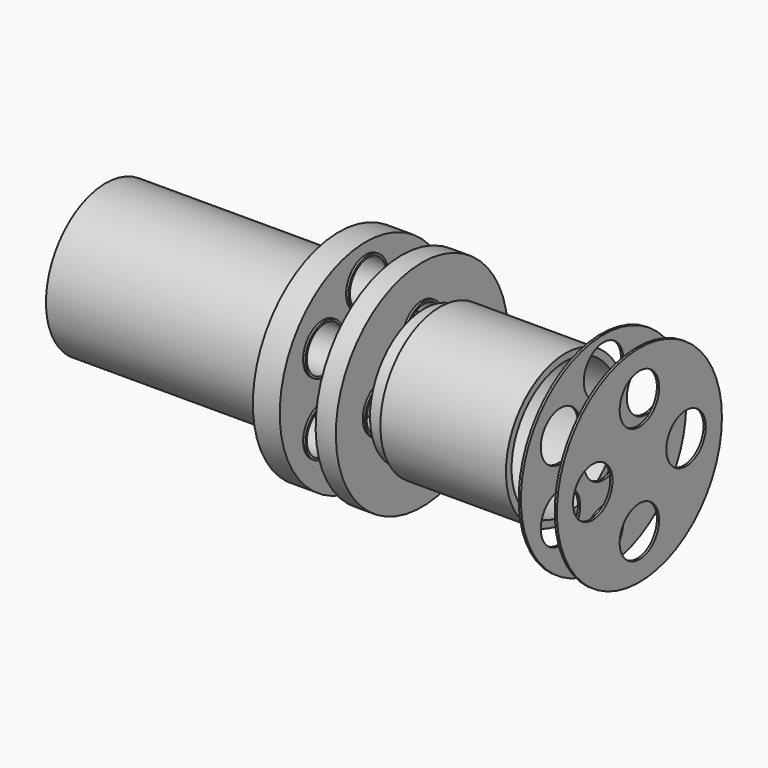
from build123d import *

# Parameters (mm, degrees)
F0_W            = 25.4
F0_H            = 47.9171
F2_R            = 52.9171
F2_R_2          = 47.9171
F3_DEPTH        = 152.4
F5_R            = 76.2
F5_R_2          = 17.4625
F7_DEPTH        = 1.5875
F8_R            = 76.2
F8_R_2          = 73.152
F9_DEPTH        = 17.4625
F10_R           = 73.152
F10_R_2         = 17.4625
F11_DEPTH       = 1.5875
F12_R           = 17.4625
F12_R_2         = 16.0655
F13_DEPTH       = 1.5875
F13_DEPTH_BACK  = 20.6375
F15_D           = 10.16
F15_CBORE_D     = 19.05
F15_CBORE_DEPTH = 12.7
F20_R           = 16.0655
F21_DEPTH       = 14.2875
F20_R_2         = 17.4625
F22_DEPTH       = 1.5875
F22_DEPTH_BACK  = 15.875
F23_W           = 88.9
F23_H           = 4.9784
F26_R           = 73.152
F26_R_2         = 17.4625
F27_DEPTH       = 1.5875
F29_R           = 73.025
F29_R_2         = 17.4625
F30_DEPTH       = 1.5875


# Not quite as in the source:
# - a length typed as a fraction of an inch, garbled in the dataset ("3 / 203.2 mm" for 3/8 in), is restored
# - a feature names something its author has since deleted; it is built from what else it names
# - the program builds the solid bodies; features that only make, move or delete a surface that nothing else refers to are left out


with BuildPart() as f1:
    # F0 (on Front) → F1 (revolve)
    with BuildSketch(Plane.XZ):
        with Locations((38.1, 23.95855)):
            Rectangle(F0_W, F0_H)
    revolve(axis=Axis((-5.279654984, 0, 0), (1, 0, 0)))

    # F15 (through all)
    with Locations(Plane(origin=(25.4, 0, 0), x_dir=(0, -1, 0), z_dir=(-1, 0, 0))):
        with Locations((0, 0)):
            CounterBoreHole(F15_D / 2, F15_CBORE_D / 2, F15_CBORE_DEPTH)


with BuildPart() as f3:
    # F2 (on face) → F3 (new body)
    with BuildSketch(Plane.YZ.offset(50.8)):
        Circle(F2_R)
        Circle(F2_R_2, mode=Mode.SUBTRACT)
    extrude(amount=-F3_DEPTH)


with BuildPart() as f7:
    # F5 (on offset) → F7 (new body)
    with BuildSketch(Plane.YZ.offset(63.5)):
        Circle(F5_R)
        with Locations((-38.1, -25.4)):
            Circle(F5_R_2, mode=Mode.SUBTRACT)
        with Locations((0, -50.8)):
            Circle(F5_R_2, mode=Mode.SUBTRACT)
        with Locations((38.1, -25.4)):
            Circle(F5_R_2, mode=Mode.SUBTRACT)
        with Locations((-38.1, 25.4)):
            Circle(F5_R_2, mode=Mode.SUBTRACT)
        Circle(F5_R_2, mode=Mode.SUBTRACT)
        with Locations((38.1, 25.4)):
            Circle(F5_R_2, mode=Mode.SUBTRACT)
        with Locations((0, 50.8)):
            Circle(F5_R_2, mode=Mode.SUBTRACT)
    extrude(amount=F7_DEPTH)

    # F8 (on face) → F9 (join)
    with BuildSketch(Plane.YZ.offset(65.0875)):
        Circle(F8_R)
        Circle(F8_R_2, mode=Mode.SUBTRACT)
    extrude(amount=F9_DEPTH)

    # F10 (on face) → F11 (join)
    with BuildSketch(Plane.YZ.offset(82.55)):
        Circle(F10_R)
        with Locations((-38.1, -25.4)):
            Circle(F10_R_2, mode=Mode.SUBTRACT)
        with Locations((0, -50.8)):
            Circle(F10_R_2, mode=Mode.SUBTRACT)
        with Locations((38.1, -25.4)):
            Circle(F10_R_2, mode=Mode.SUBTRACT)
        with Locations((-38.1, 25.4)):
            Circle(F10_R_2, mode=Mode.SUBTRACT)
        Circle(F10_R_2, mode=Mode.SUBTRACT)
        with Locations((38.1, 25.4)):
            Circle(F10_R_2, mode=Mode.SUBTRACT)
        with Locations((0, 50.8)):
            Circle(F10_R_2, mode=Mode.SUBTRACT)
    extrude(amount=-F11_DEPTH)

    # F12 (on face) → F13 (join, two sides)
    with BuildSketch(Plane.YZ.offset(82.55)) as f13_sk:
        Circle(F12_R)
        Circle(F12_R_2, mode=Mode.SUBTRACT)
        with Locations((-38.1, 25.4)):
            Circle(F12_R)
        with Locations((-38.1, 25.4)):
            Circle(F12_R_2, mode=Mode.SUBTRACT)
        with Locations((0, 50.8)):
            Circle(F12_R)
        with Locations((0, 50.8)):
            Circle(F12_R_2, mode=Mode.SUBTRACT)
        with Locations((38.1, 25.4)):
            Circle(F12_R)
        with Locations((38.1, 25.4)):
            Circle(F12_R_2, mode=Mode.SUBTRACT)
        with Locations((38.1, -25.4)):
            Circle(F12_R)
        with Locations((38.1, -25.4)):
            Circle(F12_R_2, mode=Mode.SUBTRACT)
        with Locations((0, -50.8)):
            Circle(F12_R)
        with Locations((0, -50.8)):
            Circle(F12_R_2, mode=Mode.SUBTRACT)
        with Locations((-38.1, -25.4)):
            Circle(F12_R)
        with Locations((-38.1, -25.4)):
            Circle(F12_R_2, mode=Mode.SUBTRACT)
    extrude(amount=F13_DEPTH)
    extrude(f13_sk.sketch, amount=-F13_DEPTH_BACK)


with BuildPart() as f17_1:
    # F17: instance of F1
    add(f1.part.mirror(Plane.YZ.offset(87.3125)))


with BuildPart() as f19:
    # F18 (on Front) → F19 (revolve)
    with BuildSketch(Plane.XZ):
        Polygon((107.95, 76.2), (107.95, 0), (109.5375, 0), (109.5375, 73.025), (120.65, 73.025), (120.65, 0), (122.2375, 0), (122.2375, 76.2), align=None)
    revolve(axis=Axis((197.1038290552, 0, 0), (1, 0, 0)))

    # F20 (on face) → F21 (cut, through all)
    with BuildSketch(Plane.YZ.offset(122.2375)):
        with Locations((0, 34.925)):
            Circle(F20_R)
        with Locations((-34.925, 0)):
            Circle(F20_R)
        with Locations((0, -34.925)):
            Circle(F20_R)
        with Locations((34.925, 0)):
            Circle(F20_R)
    extrude(amount=-F21_DEPTH, mode=Mode.SUBTRACT)

    # F20 (on face) → F22 (join, two sides)
    with BuildSketch(Plane.YZ.offset(122.2375)) as f22_sk:
        with Locations((0, 34.925)):
            Circle(F20_R_2)
        with Locations((0, 34.925)):
            Circle(F20_R, mode=Mode.SUBTRACT)
        with Locations((34.925, 0)):
            Circle(F20_R_2)
        with Locations((34.925, 0)):
            Circle(F20_R, mode=Mode.SUBTRACT)
        with Locations((0, -34.925)):
            Circle(F20_R_2)
        with Locations((0, -34.925)):
            Circle(F20_R, mode=Mode.SUBTRACT)
        with Locations((-34.925, 0)):
            Circle(F20_R_2)
        with Locations((-34.925, 0)):
            Circle(F20_R, mode=Mode.SUBTRACT)
    extrude(amount=F22_DEPTH)
    extrude(f22_sk.sketch, amount=-F22_DEPTH_BACK)


with BuildPart() as f24:
    # F23 (on Front) → F24 (revolve)
    with BuildSketch(Plane.XZ):
        with Locations((179.3875, 50.165)):
            Rectangle(F23_W, F23_H)
    revolve(axis=Axis((95.0557777543, 0, 0), (-1, 0, 0)))


with BuildPart() as f27:
    # F26 (on offset) → F27 (new body)
    with BuildSketch(Plane.YZ.offset(249.2375)):
        Circle(F26_R)
        with Locations((-38.1, -25.4)):
            Circle(F26_R_2, mode=Mode.SUBTRACT)
        with Locations((0, -50.8)):
            Circle(F26_R_2, mode=Mode.SUBTRACT)
        with Locations((38.1, -25.4)):
            Circle(F26_R_2, mode=Mode.SUBTRACT)
        with Locations((-38.1, 25.4)):
            Circle(F26_R_2, mode=Mode.SUBTRACT)
        Circle(F26_R_2, mode=Mode.SUBTRACT)
        with Locations((38.1, 25.4)):
            Circle(F26_R_2, mode=Mode.SUBTRACT)
        with Locations((0, 50.8)):
            Circle(F26_R_2, mode=Mode.SUBTRACT)
    extrude(amount=F27_DEPTH)


with BuildPart() as f30:
    # F29 (on offset) → F30 (new body)
    with BuildSketch(Plane.YZ.offset(274.6375)):
        Circle(F29_R)
        with Locations((0, -41.275)):
            Circle(F29_R_2, mode=Mode.SUBTRACT)
        with Locations((-41.275, 0)):
            Circle(F29_R_2, mode=Mode.SUBTRACT)
        with Locations((41.275, 0)):
            Circle(F29_R_2, mode=Mode.SUBTRACT)
        with Locations((0, 41.275)):
            Circle(F29_R_2, mode=Mode.SUBTRACT)
    extrude(amount=F30_DEPTH)


solid = Compound([f1.part, f3.part, f7.part, f17_1.part, f19.part, f24.part, f27.part, f30.part])
